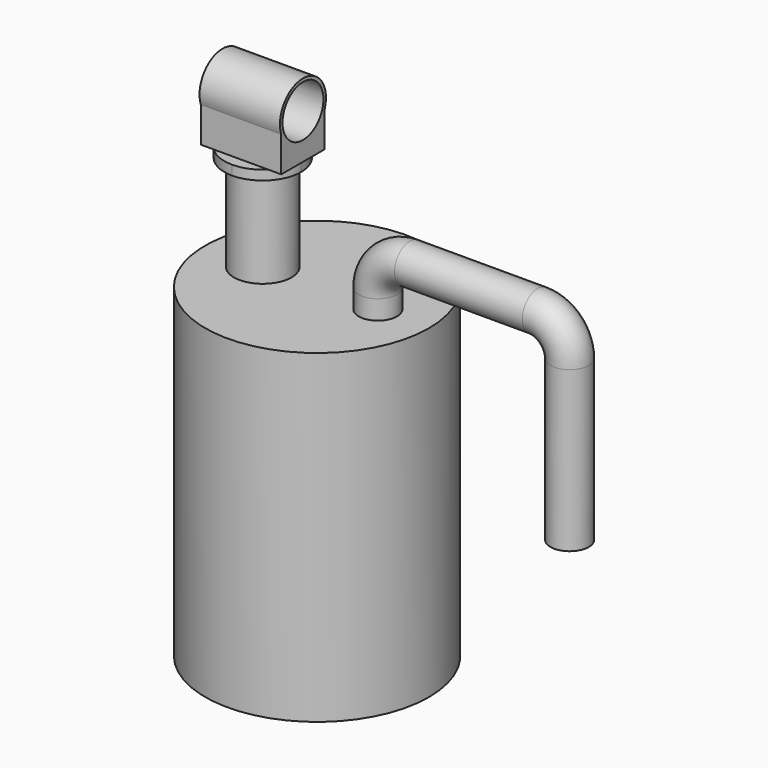
from build123d import *

# Parameters (mm, degrees)
F0_R      = 175
F0_R_2    = 172
F1_DEPTH  = 500
F2_DEPTH  = 4
F3_R      = 175
F3_R_2    = 172
F4_DEPTH  = 4
F5_R      = 30
F5_R_2    = 25
F5_R_3    = 45
F5_R_4    = 40
F11_DEPTH = 15
F13_R     = 39.999999
F14_DEPTH = 62.9


with BuildPart() as f1:
    # F0 (on Top) → F1 (new body)
    with BuildSketch(Plane.XY):
        Circle(F0_R)
        Circle(F0_R_2, mode=Mode.SUBTRACT)
    extrude(amount=F1_DEPTH)

    # F0 (on Top) → F2 (join)
    with BuildSketch(Plane.XY):
        Circle(F0_R)
        Circle(F0_R_2, mode=Mode.SUBTRACT)
        Circle(F0_R_2)
    extrude(amount=-F2_DEPTH)

    # F3 (on face) → F4 (join)
    with BuildSketch(Plane.XY.offset(500)):
        Circle(F3_R)
        Circle(F3_R_2, mode=Mode.SUBTRACT)
        Circle(F3_R_2)
    extrude(amount=F4_DEPTH)

    # F8: sweep along a path in F7
    with BuildLine(Plane(origin=(0, 0, 0), x_dir=(-1, 0, 0), z_dir=(0, 1, 0))) as f8_path:
        Line((-95, 504), (-95, 534))
        ThreePointArc((-95, 534), (-109.644661, 569.355339), (-145, 584))
        Line((-145, 584), (-345, 584))
        ThreePointArc((-345, 584), (-380.355339, 569.355339), (-395, 534))
        Line((-395, 534), (-395, 284))
    # F5 (on face) → F8 (sweep)
    with BuildSketch(Plane.XY.offset(504)):
        with Locations((95, 0)):
            Circle(F5_R)
        with Locations((95, 0)):
            Circle(F5_R_2, mode=Mode.SUBTRACT)
    sweep(path=f8_path.line)

    # F9: sweep along a path in F7
    with BuildLine(Plane(origin=(0, 0, 0), x_dir=(-1, 0, 0), z_dir=(0, 1, 0))) as f9_path:
        Line((85, 504), (85, 654))
    # F5 (on face) → F9 (sweep)
    with BuildSketch(Plane.XY.offset(504)):
        with Locations((-85, 0)):
            Circle(F5_R_3)
        with Locations((-85, 0)):
            Circle(F5_R_4, mode=Mode.SUBTRACT)
    sweep(path=f9_path.line)

    # F10 (on face) → F11 (join)
    with BuildSketch(Plane.XY.offset(654)):
        with BuildLine():
            ThreePointArc((-25, 0), (-127.426407, 42.426407), (-85, -60))
            ThreePointArc((-85, -60), (-42.573593, -42.426407), (-25, 0))
        make_face()
        with BuildLine():
            ThreePointArc((-85, -45), (-116.819805, 31.819805), (-40, 0))
            ThreePointArc((-40, 0), (-53.180195, -31.819805), (-85, -45))
        make_face(mode=Mode.SUBTRACT)
        with BuildLine():
            ThreePointArc((-85, -45), (-53.180195, -31.819805), (-40, 0))
            ThreePointArc((-40, 0), (-116.819805, 31.819805), (-85, -45))
        make_face()
        with BuildLine():
            ThreePointArc((-45, 0), (-56.715729, -28.284271), (-85, -40))
            ThreePointArc((-85, -40), (-113.284271, 28.284271), (-45, 0))
        make_face(mode=Mode.SUBTRACT)
    extrude(amount=F11_DEPTH)

    # F13 (on line) → F14 (join, symmetric)
    with BuildSketch(Plane.YZ.offset(-85)):
        with BuildLine():
            ThreePointArc((42.5, 724.209801), (0, 694), (-42.5, 724.209801))
            Line((-42.5, 724.209801), (-42.5, 669))
            Line((-42.5, 669), (42.5, 669))
            Line((42.5, 669), (42.5, 724.209801))
        make_face()
        with BuildLine():
            ThreePointArc((42.5, 724.209801), (44.370598, 731.5), (45, 739))
            ThreePointArc((45, 739), (-7.5, 783.370598), (-42.5, 724.209801))
            ThreePointArc((-42.5, 724.209801), (0, 694), (42.5, 724.209801))
        make_face()
        with Locations((0, 739)):
            Circle(F13_R, mode=Mode.SUBTRACT)
    extrude(amount=F14_DEPTH, both=True)


solid = f1.part
